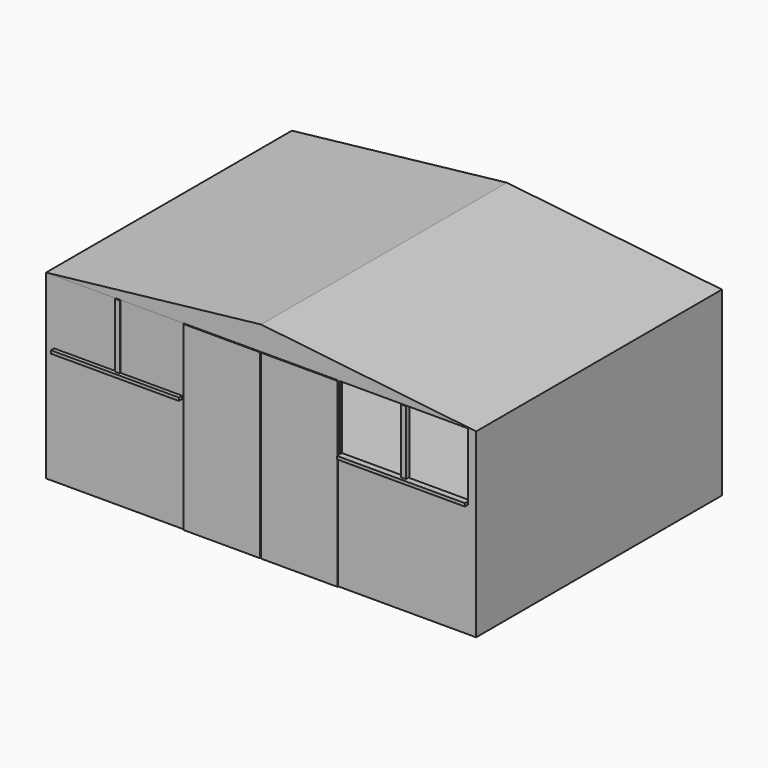
from build123d import *

# Parameters (mm, degrees)
F0_W          = 427
F0_H          = 305
F0_W_2        = 422.6
F0_H_2        = 300.6
F1_DEPTH      = 180
F2_DEPTH      = 2.2
F3_W          = 76
F3_H          = 180
F3_W_2        = 5
F3_H_2        = 63.7124854326
F4_DEPTH      = 1
F4_DEPTH_BACK = 3.3
F3_W_3        = 61
F5_DEPTH      = 25
F6_DEPTH      = 8
F7_DEPTH      = 4
F9_DEPTH      = 305


# Not quite as in the source:
# - a feature names something its author has since deleted; it is built from what else it names
# - the program builds the solid bodies; features that only make, move or delete a surface that nothing else refers to are left out


with BuildPart() as f1:
    # F0 (on Top) → F1 (new body)
    with BuildSketch(Plane.XY):
        with Locations((213.5, -152.5)):
            Rectangle(F0_W, F0_H)
        with Locations((213.5, -152.5)):
            Rectangle(F0_W_2, F0_H_2, mode=Mode.SUBTRACT)
    extrude(amount=F1_DEPTH)

    # F0 (on Top) → F2 (join)
    with BuildSketch(Plane.XY):
        with Locations((213.5, -152.5)):
            Rectangle(F0_W_2, F0_H_2)
    extrude(amount=F2_DEPTH)

    # F3 (on face) → F4 (join, two sides)
    with BuildSketch(Plane.XZ.offset(305)) as f4_sk:
        with Locations((175, 90)):
            Rectangle(F3_W, F3_H)
        with Locations((252, 90)):
            Rectangle(F3_W, F3_H)
        with Locations((71.5, 148.1437572837)):
            Rectangle(F3_W_2, F3_H_2)
        with Locations((355.5, 148.1437572837)):
            Rectangle(F3_W_2, F3_H_2)
    extrude(amount=F4_DEPTH)
    extrude(f4_sk.sketch, amount=-F4_DEPTH_BACK)

    # F3 (on face) → F5 (cut)
    with BuildSketch(Plane.XZ.offset(305)):
        Polygon((135, 180), (137, 180), (213, 180), (214, 180), (290, 180), (292, 180), (353, 180), (358, 180), (419, 180), (427, 180), (213.5, 204), (0, 180), (8, 180), (69, 180), (74, 180), align=None)
        with Locations((322.5, 148.1437572837)):
            Rectangle(F3_W_3, F3_H_2)
        with Locations((388.5, 148.1437572837)):
            Rectangle(F3_W_3, F3_H_2)
    extrude(amount=-F5_DEPTH, mode=Mode.SUBTRACT)

    # F3 (on face) → F6 (join)
    with BuildSketch(Plane.XZ.offset(305)):
        Polygon((135, 180), (137, 180), (213, 180), (214, 180), (290, 180), (292, 180), (353, 180), (358, 180), (419, 180), (427, 180), (213.5, 204), (0, 180), (8, 180), (69, 180), (74, 180), align=None)
    extrude(amount=-F6_DEPTH)

    # F3 (on face) → F7 (join)
    with BuildSketch(Plane.XZ.offset(305)):
        Polygon((353, 116.2875145674), (292, 116.2875145674), (292, 113.2875145674), (419, 113.2875145674), (419, 116.2875145674), (358, 116.2875145674), align=None)
        Polygon((135, 113.2875145674), (135, 116.2875145674), (74, 116.2875145674), (69, 116.2875145674), (8, 116.2875145674), (8, 113.2875145674), align=None)
    extrude(amount=F7_DEPTH)


with BuildPart() as f9:
    # F8 (on face) → F9 (new body)
    with BuildSketch(Plane(origin=(0, 0, 0), x_dir=(-1, 0, 0), z_dir=(0, 1, 0))):
        Polygon((-213.5, 204), (-427, 180), (0, 180), align=None)
    extrude(amount=-F9_DEPTH)


solid = Compound([f1.part, f9.part])
